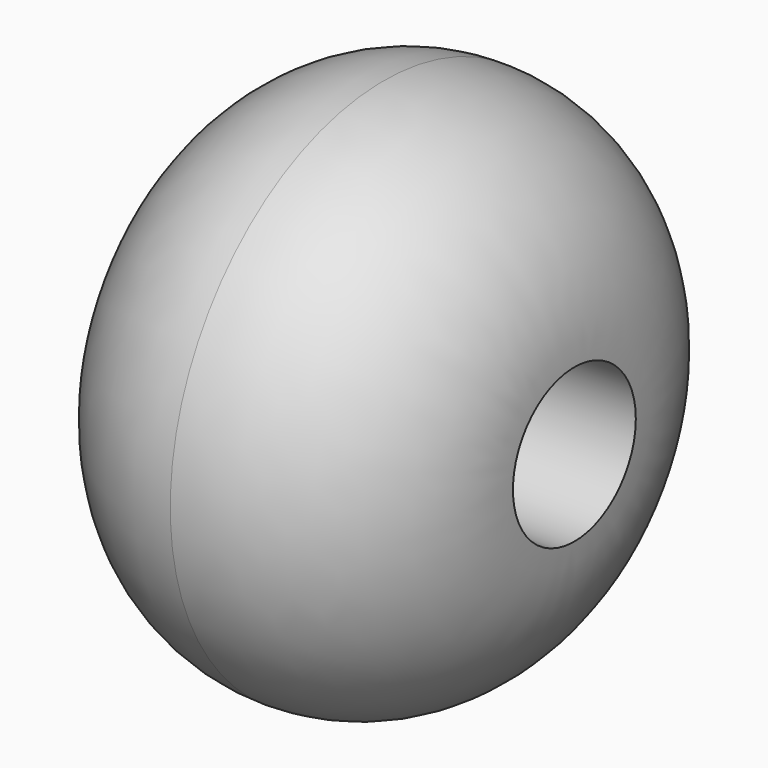
from build123d import *

# Parameters (mm, degrees)
F0_R     = 17.5428851577
F1_DEPTH = 25
F2_R     = 12.5
F3_R     = 12.49999
F4_DEPTH = 25.001


# Not quite as in the source:
# - a fillet or chamfer is up to 0.001 mm smaller than in the source, because OpenCascade refuses the exact size


with BuildPart() as f1:
    # F0 (on Right) → F1 (new body)
    with BuildSketch(Plane.YZ):
        with Locations((-25.815801695, -30.2766188979)):
            Circle(F0_R)
    extrude(amount=F1_DEPTH)

    # F2
    f2_edges = [f1.edges().sort_by_distance(p)[0] for p in [
        (25, -43.358687, -30.276619),
    ]]
    fillet(f2_edges, radius=F2_R)

    # F3 (radius 12.5 in the source; OpenCascade refuses exactly that, so slightly less here)
    f3_edges = [f1.edges().sort_by_distance(p)[0] for p in [
        (0, -43.358687, -30.276619),
    ]]
    fillet(f3_edges, radius=F3_R)

    # F4 (cut, through all): a face of the model
    f4_faces = [f1.faces().sort_by_distance(p)[0] for p in [
        (25, -25.815801695, -30.2766188979),
    ]]
    extrude(f4_faces, amount=-F4_DEPTH, mode=Mode.SUBTRACT)


solid = f1.part
